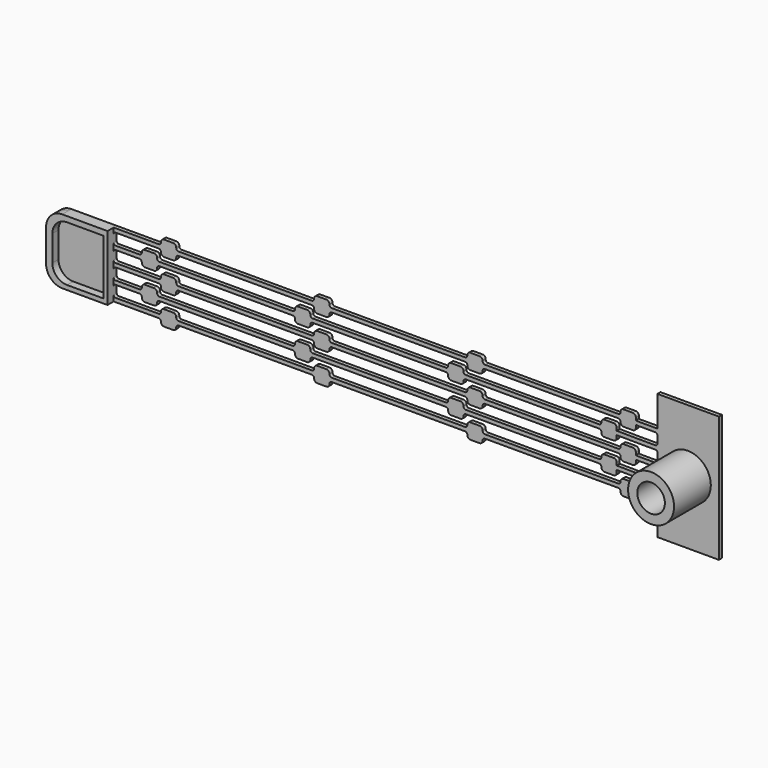
from build123d import *

# Parameters (mm, degrees)
F1_DEPTH = 0.25
F3_DEPTH = 0.5
F5_DEPTH = 0.5
F6_R     = 1.5
F6_R_2   = 0.9
F7_DEPTH = 3


# Not quite as in the source:
# - ends of sketch curves that miss each other by under 0.0002 mm in the source are joined


with BuildPart() as f1:
    # F0 (on Front) → F1 (new body)
    with BuildSketch(Plane.XZ):
        with BuildLine():
            Line((49.9212476134, 27.0172210783), (50.5212476134, 27.0172210783))
            ThreePointArc((50.5212476134, 27.0172210783), (50.6626689697, 27.075799722), (50.7212476134, 27.2172210783))
            Line((50.7212476134, 27.2172210783), (50.7212476134, 27.2422210783))
            ThreePointArc((50.7212476134, 27.2422210783), (50.7651815963, 27.3482870955), (50.8712476134, 27.3922210783))
            Line((50.8712476134, 27.3922210783), (51.1654019356, 27.3922210783))
            Line((51.1654019356, 27.3922210783), (57.8865653276, 27.3922210783))
            Line((57.8865653276, 27.3922210783), (59.1332476134, 27.3922210783))
            Line((59.1332476134, 27.3922210783), (59.5712476134, 27.3922210783))
            ThreePointArc((59.5712476134, 27.3922210783), (59.6773136306, 27.3482870955), (59.7212476134, 27.2422210783))
            Line((59.7212476134, 27.2422210783), (59.7212476134, 27.2172210783))
            ThreePointArc((59.7212476134, 27.2172210783), (59.7798262572, 27.075799722), (59.9212476134, 27.0172210783))
            Line((59.9212476134, 27.0172210783), (60.5212476134, 27.0172210783))
            ThreePointArc((60.5212476134, 27.0172210783), (60.6626689697, 27.075799722), (60.7212476134, 27.2172210783))
            Line((60.7212476134, 27.2172210783), (60.7212476134, 27.2422210783))
            ThreePointArc((60.7212476134, 27.2422210783), (60.7651815963, 27.3482870955), (60.8712476134, 27.3922210783))
            Line((60.8712476134, 27.3922210783), (61.1654019356, 27.3922210783))
            Line((61.1654019356, 27.3922210783), (67.8865653276, 27.3922210783))
            Line((67.8865653276, 27.3922210783), (69.1332476134, 27.3922210783))
            Line((69.1332476134, 27.3922210783), (69.5712476134, 27.3922210783))
            ThreePointArc((69.5712476134, 27.3922210783), (69.6773136306, 27.3482870955), (69.7212476134, 27.2422210783))
            Line((69.7212476134, 27.2422210783), (69.7212476134, 27.2172210783))
            ThreePointArc((69.7212476134, 27.2172210783), (69.7798262572, 27.075799722), (69.9212476134, 27.0172210783))
            Line((69.9212476134, 27.0172210783), (70.5212476134, 27.0172210783))
            ThreePointArc((70.5212476134, 27.0172210783), (70.6626689697, 27.075799722), (70.7212476134, 27.2172210783))
            Line((70.7212476134, 27.2172210783), (70.7212476134, 27.2422210783))
            ThreePointArc((70.7212476134, 27.2422210783), (70.7651815963, 27.3482870955), (70.8712476134, 27.3922210783))
            Line((70.8712476134, 27.3922210783), (71.1654019356, 27.3922210783))
            Line((71.1654019356, 27.3922210783), (77.8865653276, 27.3922210783))
            Line((77.8865653276, 27.3922210783), (79.1332476134, 27.3922210783))
            Line((79.1332476134, 27.3922210783), (79.5712476134, 27.3922210783))
            ThreePointArc((79.5712476134, 27.3922210783), (79.6773136306, 27.3482870955), (79.7212476134, 27.2422210783))
            Line((79.7212476134, 27.2422210783), (79.7212476134, 27.2172210783))
            ThreePointArc((79.7212476134, 27.2172210783), (79.7798262572, 27.075799722), (79.9212476134, 27.0172210783))
            Line((79.9212476134, 27.0172210783), (80.5212476134, 27.0172210783))
            ThreePointArc((80.5212476134, 27.0172210783), (80.6626689697, 27.075799722), (80.7212476134, 27.2172210783))
            Line((80.7212476134, 27.2172210783), (80.7212476134, 27.2422210783))
            Line((80.7212476134, 27.2422210783), (80.7212476134, 27.3922210783))
            Line((80.7212476134, 27.3922210783), (80.8795653284, 27.3786683083))
            Line((80.8795653284, 27.3786683083), (82.1295653284, 27.3786683083))
            Line((82.1295653284, 27.3786683083), (82.1295653284, 25.3928024322))
            Line((82.1295653284, 25.3928024322), (86.1411392689, 25.3928024322))
            Line((86.1411392689, 25.3928024322), (86.1411392689, 27.3786683083))
            Line((86.1411392689, 27.3786683083), (86.1411392689, 28.4439172033))
            Line((86.1411392689, 28.4439172033), (86.1411392689, 30.5634194132))
            Line((86.1411392689, 30.5634194132), (86.1411392689, 31.6286683083))
            Line((86.1411392689, 31.6286683083), (86.1411392689, 33.6259715259))
            Line((86.1411392689, 33.6259715259), (82.1295653284, 33.6259715259))
            Line((82.1295653284, 33.6259715259), (82.1295653284, 31.6286683083))
            Line((82.1295653284, 31.6286683083), (80.8795653284, 31.6286683083))
            Line((80.8795653284, 31.6286683083), (80.7212476134, 31.6422210783))
            Line((80.7212476134, 31.6422210783), (80.7212476134, 31.7922210783))
            Line((80.7212476134, 31.7922210783), (80.7212476134, 31.8172210783))
            ThreePointArc((80.7212476134, 31.8172210783), (80.6626689697, 31.9586424345), (80.5212476134, 32.0172210783))
            Line((80.5212476134, 32.0172210783), (79.9212476134, 32.0172210783))
            ThreePointArc((79.9212476134, 32.0172210783), (79.7798262572, 31.9586424345), (79.7212476134, 31.8172210783))
            Line((79.7212476134, 31.8172210783), (79.7212476134, 31.7922210783))
            ThreePointArc((79.7212476134, 31.7922210783), (79.6773136306, 31.6861550611), (79.5712476134, 31.6422210783))
            Line((79.5712476134, 31.6422210783), (79.1332476134, 31.6422210783))
            Line((79.1332476134, 31.6422210783), (77.8865653276, 31.6422210783))
            Line((77.8865653276, 31.6422210783), (71.1654019356, 31.6422210783))
            Line((71.1654019356, 31.6422210783), (70.8712476134, 31.6422210783))
            ThreePointArc((70.8712476134, 31.6422210783), (70.7651815963, 31.6861550611), (70.7212476134, 31.7922210783))
            Line((70.7212476134, 31.7922210783), (70.7212476134, 31.8172210783))
            ThreePointArc((70.7212476134, 31.8172210783), (70.6626689697, 31.9586424345), (70.5212476134, 32.0172210783))
            Line((70.5212476134, 32.0172210783), (69.9212476134, 32.0172210783))
            ThreePointArc((69.9212476134, 32.0172210783), (69.7798262572, 31.9586424345), (69.7212476134, 31.8172210783))
            Line((69.7212476134, 31.8172210783), (69.7212476134, 31.7922210783))
            ThreePointArc((69.7212476134, 31.7922210783), (69.6773136306, 31.6861550611), (69.5712476134, 31.6422210783))
            Line((69.5712476134, 31.6422210783), (69.1332476134, 31.6422210783))
            Line((69.1332476134, 31.6422210783), (67.8865653276, 31.6422210783))
            Line((67.8865653276, 31.6422210783), (61.1654019356, 31.6422210783))
            Line((61.1654019356, 31.6422210783), (60.8712476134, 31.6422210783))
            ThreePointArc((60.8712476134, 31.6422210783), (60.7651815963, 31.6861550611), (60.7212476134, 31.7922210783))
            Line((60.7212476134, 31.7922210783), (60.7212476134, 31.8172210783))
            ThreePointArc((60.7212476134, 31.8172210783), (60.6626689697, 31.9586424345), (60.5212476134, 32.0172210783))
            Line((60.5212476134, 32.0172210783), (59.9212476134, 32.0172210783))
            ThreePointArc((59.9212476134, 32.0172210783), (59.7798262572, 31.9586424345), (59.7212476134, 31.8172210783))
            Line((59.7212476134, 31.8172210783), (59.7212476134, 31.7922210783))
            ThreePointArc((59.7212476134, 31.7922210783), (59.6773136306, 31.6861550611), (59.5712476134, 31.6422210783))
            Line((59.5712476134, 31.6422210783), (59.1332476134, 31.6422210783))
            Line((59.1332476134, 31.6422210783), (57.8865653276, 31.6422210783))
            Line((57.8865653276, 31.6422210783), (51.1654019356, 31.6422210783))
            Line((51.1654019356, 31.6422210783), (50.8712476134, 31.6422210783))
            ThreePointArc((50.8712476134, 31.6422210783), (50.7651815963, 31.6861550611), (50.7212476134, 31.7922210783))
            Line((50.7212476134, 31.7922210783), (50.7212476134, 31.8172210783))
            ThreePointArc((50.7212476134, 31.8172210783), (50.6626689697, 31.9586424345), (50.5212476134, 32.0172210783))
            Line((50.5212476134, 32.0172210783), (49.9212476134, 32.0172210783))
            ThreePointArc((49.9212476134, 32.0172210783), (49.7798262572, 31.9586424345), (49.7212476134, 31.8172210783))
            Line((49.7212476134, 31.8172210783), (49.7212476134, 31.7922210783))
            ThreePointArc((49.7212476134, 31.7922210783), (49.6773136306, 31.6861550611), (49.5712476134, 31.6422210783))
            Line((49.5712476134, 31.6422210783), (49.1332476134, 31.6422210783))
            Line((49.1332476134, 31.6422210783), (47.8865653276, 31.6422210783))
            Line((47.8865653276, 31.6422210783), (43.6902402822, 31.6422210783))
            ThreePointArc((43.6902402822, 31.6422210783), (42.9369955648, 31.3302169006), (42.6249913871, 30.5769721832))
            Line((42.6249913871, 30.5769721832), (42.6249913871, 28.4574699733))
            ThreePointArc((42.6249913871, 28.4574699733), (42.9369955648, 27.704225256), (43.6902402822, 27.3922210783))
            Line((43.6902402822, 27.3922210783), (47.8865653276, 27.3922210783))
            Line((47.8865653276, 27.3922210783), (49.1332476134, 27.3922210783))
            Line((49.1332476134, 27.3922210783), (49.5712476134, 27.3922210783))
            ThreePointArc((49.5712476134, 27.3922210783), (49.6773136306, 27.3482870955), (49.7212476134, 27.2422210783))
            Line((49.7212476134, 27.2422210783), (49.7212476134, 27.2172210783))
            ThreePointArc((49.7212476134, 27.2172210783), (49.7798262572, 27.075799722), (49.9212476134, 27.0172210783))
        make_face()
        with BuildLine():
            ThreePointArc((50.7212476134, 27.8172210783), (50.6626689697, 27.9586424345), (50.5212476134, 28.0172210783))
            Line((50.5212476134, 28.0172210783), (49.9212476134, 28.0172210783))
            ThreePointArc((49.9212476134, 28.0172210783), (49.7798262572, 27.9586424345), (49.7212476134, 27.8172210783))
            Line((49.7212476134, 27.8172210783), (49.7212476134, 27.7922210783))
            ThreePointArc((49.7212476134, 27.7922210783), (49.6773136306, 27.6861550611), (49.5712476134, 27.6422210783))
            Line((49.5712476134, 27.6422210783), (49.1332476134, 27.6422210783))
            Line((49.1332476134, 27.6422210783), (47.8865653276, 27.6422210783))
            Line((47.8865653276, 27.6422210783), (46.7647824857, 27.6422210783))
            ThreePointArc((46.7647824857, 27.6422210783), (46.6741192638, 27.6797750144), (46.6365653276, 27.7704382363))
            Line((46.6365653276, 27.7704382363), (46.6365653276, 28.2640039202))
            ThreePointArc((46.6365653276, 28.2640039202), (46.6741192638, 28.3546671421), (46.7647824857, 28.3922210783))
            Line((46.7647824857, 28.3922210783), (47.8865653276, 28.3922210783))
            Line((47.8865653276, 28.3922210783), (48.3212476134, 28.3922210783))
            ThreePointArc((48.3212476134, 28.3922210783), (48.4273136306, 28.3482870955), (48.4712476134, 28.2422210783))
            Line((48.4712476134, 28.2422210783), (48.4712476134, 28.2172210783))
            ThreePointArc((48.4712476134, 28.2172210783), (48.5298262572, 28.075799722), (48.6712476134, 28.0172210783))
            Line((48.6712476134, 28.0172210783), (49.2712476134, 28.0172210783))
            ThreePointArc((49.2712476134, 28.0172210783), (49.4126689697, 28.075799722), (49.4712476134, 28.2172210783))
            Line((49.4712476134, 28.2172210783), (49.4712476134, 28.2422210783))
            ThreePointArc((49.4712476134, 28.2422210783), (49.5151815963, 28.3482870955), (49.6212476134, 28.3922210783))
            Line((49.6212476134, 28.3922210783), (51.1654019356, 28.3922210783))
            Line((51.1654019356, 28.3922210783), (57.8865653276, 28.3922210783))
            Line((57.8865653276, 28.3922210783), (58.3212476134, 28.3922210783))
            ThreePointArc((58.3212476134, 28.3922210783), (58.4273136306, 28.3482870955), (58.4712476134, 28.2422210783))
            Line((58.4712476134, 28.2422210783), (58.4712476134, 28.2172210783))
            ThreePointArc((58.4712476134, 28.2172210783), (58.5298262572, 28.075799722), (58.6712476134, 28.0172210783))
            Line((58.6712476134, 28.0172210783), (59.2712476134, 28.0172210783))
            ThreePointArc((59.2712476134, 28.0172210783), (59.4126689697, 28.075799722), (59.4712476134, 28.2172210783))
            Line((59.4712476134, 28.2172210783), (59.4712476134, 28.2422210783))
            ThreePointArc((59.4712476134, 28.2422210783), (59.5151815963, 28.3482870955), (59.6212476134, 28.3922210783))
            Line((59.6212476134, 28.3922210783), (61.1654019356, 28.3922210783))
            Line((61.1654019356, 28.3922210783), (67.8865653276, 28.3922210783))
            Line((67.8865653276, 28.3922210783), (68.3212476134, 28.3922210783))
            ThreePointArc((68.3212476134, 28.3922210783), (68.4273136306, 28.3482870955), (68.4712476134, 28.2422210783))
            Line((68.4712476134, 28.2422210783), (68.4712476134, 28.2172210783))
            ThreePointArc((68.4712476134, 28.2172210783), (68.5298262572, 28.075799722), (68.6712476134, 28.0172210783))
            Line((68.6712476134, 28.0172210783), (69.2712476134, 28.0172210783))
            ThreePointArc((69.2712476134, 28.0172210783), (69.4126689697, 28.075799722), (69.4712476134, 28.2172210783))
            Line((69.4712476134, 28.2172210783), (69.4712476134, 28.2422210783))
            ThreePointArc((69.4712476134, 28.2422210783), (69.5151815963, 28.3482870955), (69.6212476134, 28.3922210783))
            Line((69.6212476134, 28.3922210783), (71.1654019356, 28.3922210783))
            Line((71.1654019356, 28.3922210783), (77.8865653276, 28.3922210783))
            Line((77.8865653276, 28.3922210783), (78.3212476134, 28.3922210783))
            ThreePointArc((78.3212476134, 28.3922210783), (78.4273136306, 28.3482870955), (78.4712476134, 28.2422210783))
            Line((78.4712476134, 28.2422210783), (78.4712476134, 28.2172210783))
            ThreePointArc((78.4712476134, 28.2172210783), (78.5298262572, 28.075799722), (78.6712476134, 28.0172210783))
            Line((78.6712476134, 28.0172210783), (79.2712476134, 28.0172210783))
            ThreePointArc((79.2712476134, 28.0172210783), (79.4126689697, 28.075799722), (79.4712476134, 28.2172210783))
            Line((79.4712476134, 28.2172210783), (79.4712476134, 28.2422210783))
            Line((79.4712476134, 28.2422210783), (79.4712476134, 28.3922210783))
            Line((79.4712476134, 28.3922210783), (80.8795653284, 28.3786683083))
            Line((80.8795653284, 28.3786683083), (82.0013481703, 28.3786683083))
            ThreePointArc((82.0013481703, 28.3786683083), (82.0920113922, 28.3411143721), (82.1295653284, 28.2504511502))
            Line((82.1295653284, 28.2504511502), (82.1295653284, 27.7568854663))
            ThreePointArc((82.1295653284, 27.7568854663), (82.0920113922, 27.6662222444), (82.0013481703, 27.6286683083))
            Line((82.0013481703, 27.6286683083), (80.8795653284, 27.6286683083))
            Line((80.8795653284, 27.6286683083), (80.7212476134, 27.6422210783))
            Line((80.7212476134, 27.6422210783), (80.7212476134, 27.7922210783))
            Line((80.7212476134, 27.7922210783), (80.7212476134, 27.8172210783))
            ThreePointArc((80.7212476134, 27.8172210783), (80.6626689697, 27.9586424345), (80.5212476134, 28.0172210783))
            Line((80.5212476134, 28.0172210783), (79.9212476134, 28.0172210783))
            ThreePointArc((79.9212476134, 28.0172210783), (79.7798262572, 27.9586424345), (79.7212476134, 27.8172210783))
            Line((79.7212476134, 27.8172210783), (79.7212476134, 27.7922210783))
            ThreePointArc((79.7212476134, 27.7922210783), (79.6773136306, 27.6861550611), (79.5712476134, 27.6422210783))
            Line((79.5712476134, 27.6422210783), (79.1332476134, 27.6422210783))
            Line((79.1332476134, 27.6422210783), (77.8865653276, 27.6422210783))
            Line((77.8865653276, 27.6422210783), (71.1654019356, 27.6422210783))
            Line((71.1654019356, 27.6422210783), (70.8712476134, 27.6422210783))
            ThreePointArc((70.8712476134, 27.6422210783), (70.7651815963, 27.6861550611), (70.7212476134, 27.7922210783))
            Line((70.7212476134, 27.7922210783), (70.7212476134, 27.8172210783))
            ThreePointArc((70.7212476134, 27.8172210783), (70.6626689697, 27.9586424345), (70.5212476134, 28.0172210783))
            Line((70.5212476134, 28.0172210783), (69.9212476134, 28.0172210783))
            ThreePointArc((69.9212476134, 28.0172210783), (69.7798262572, 27.9586424345), (69.7212476134, 27.8172210783))
            Line((69.7212476134, 27.8172210783), (69.7212476134, 27.7922210783))
            ThreePointArc((69.7212476134, 27.7922210783), (69.6773136306, 27.6861550611), (69.5712476134, 27.6422210783))
            Line((69.5712476134, 27.6422210783), (69.1332476134, 27.6422210783))
            Line((69.1332476134, 27.6422210783), (67.8865653276, 27.6422210783))
            Line((67.8865653276, 27.6422210783), (61.1654019356, 27.6422210783))
            Line((61.1654019356, 27.6422210783), (60.8712476134, 27.6422210783))
            ThreePointArc((60.8712476134, 27.6422210783), (60.7651815963, 27.6861550611), (60.7212476134, 27.7922210783))
            Line((60.7212476134, 27.7922210783), (60.7212476134, 27.8172210783))
            ThreePointArc((60.7212476134, 27.8172210783), (60.6626689697, 27.9586424345), (60.5212476134, 28.0172210783))
            Line((60.5212476134, 28.0172210783), (59.9212476134, 28.0172210783))
            ThreePointArc((59.9212476134, 28.0172210783), (59.7798262572, 27.9586424345), (59.7212476134, 27.8172210783))
            Line((59.7212476134, 27.8172210783), (59.7212476134, 27.7922210783))
            ThreePointArc((59.7212476134, 27.7922210783), (59.6773136306, 27.6861550611), (59.5712476134, 27.6422210783))
            Line((59.5712476134, 27.6422210783), (59.1332476134, 27.6422210783))
            Line((59.1332476134, 27.6422210783), (57.8865653276, 27.6422210783))
            Line((57.8865653276, 27.6422210783), (51.1654019356, 27.6422210783))
            Line((51.1654019356, 27.6422210783), (50.8712476134, 27.6422210783))
            ThreePointArc((50.8712476134, 27.6422210783), (50.7651815963, 27.6861550611), (50.7212476134, 27.7922210783))
            Line((50.7212476134, 27.7922210783), (50.7212476134, 27.8172210783))
        make_face(mode=Mode.SUBTRACT)
        with BuildLine():
            Line((48.3212476134, 28.6422210783), (47.8865653276, 28.6422210783))
            Line((47.8865653276, 28.6422210783), (46.7647824857, 28.6422210783))
            ThreePointArc((46.7647824857, 28.6422210783), (46.6741192638, 28.6797750144), (46.6365653276, 28.7704382363))
            Line((46.6365653276, 28.7704382363), (46.6365653276, 29.2640039202))
            ThreePointArc((46.6365653276, 29.2640039202), (46.6741192638, 29.3546671421), (46.7647824857, 29.3922210783))
            Line((46.7647824857, 29.3922210783), (47.8865653276, 29.3922210783))
            Line((47.8865653276, 29.3922210783), (49.1332476134, 29.3922210783))
            Line((49.1332476134, 29.3922210783), (49.5712476134, 29.3922210783))
            ThreePointArc((49.5712476134, 29.3922210783), (49.6773136306, 29.3482870955), (49.7212476134, 29.2422210783))
            Line((49.7212476134, 29.2422210783), (49.7212476134, 29.2172210783))
            ThreePointArc((49.7212476134, 29.2172210783), (49.7798262572, 29.075799722), (49.9212476134, 29.0172210783))
            Line((49.9212476134, 29.0172210783), (50.5212476134, 29.0172210783))
            ThreePointArc((50.5212476134, 29.0172210783), (50.6626689697, 29.075799722), (50.7212476134, 29.2172210783))
            Line((50.7212476134, 29.2172210783), (50.7212476134, 29.2422210783))
            ThreePointArc((50.7212476134, 29.2422210783), (50.7651815963, 29.3482870955), (50.8712476134, 29.3922210783))
            Line((50.8712476134, 29.3922210783), (51.1654019356, 29.3922210783))
            Line((51.1654019356, 29.3922210783), (57.8865653276, 29.3922210783))
            Line((57.8865653276, 29.3922210783), (59.1332476134, 29.3922210783))
            Line((59.1332476134, 29.3922210783), (59.5712476134, 29.3922210783))
            ThreePointArc((59.5712476134, 29.3922210783), (59.6773136306, 29.3482870955), (59.7212476134, 29.2422210783))
            Line((59.7212476134, 29.2422210783), (59.7212476134, 29.2172210783))
            ThreePointArc((59.7212476134, 29.2172210783), (59.7798262572, 29.075799722), (59.9212476134, 29.0172210783))
            Line((59.9212476134, 29.0172210783), (60.5212476134, 29.0172210783))
            ThreePointArc((60.5212476134, 29.0172210783), (60.6626689697, 29.075799722), (60.7212476134, 29.2172210783))
            Line((60.7212476134, 29.2172210783), (60.7212476134, 29.2422210783))
            ThreePointArc((60.7212476134, 29.2422210783), (60.7651815963, 29.3482870955), (60.8712476134, 29.3922210783))
            Line((60.8712476134, 29.3922210783), (61.1654019356, 29.3922210783))
            Line((61.1654019356, 29.3922210783), (67.8865653276, 29.3922210783))
            Line((67.8865653276, 29.3922210783), (69.1332476134, 29.3922210783))
            Line((69.1332476134, 29.3922210783), (69.5712476134, 29.3922210783))
            ThreePointArc((69.5712476134, 29.3922210783), (69.6773136306, 29.3482870955), (69.7212476134, 29.2422210783))
            Line((69.7212476134, 29.2422210783), (69.7212476134, 29.2172210783))
            ThreePointArc((69.7212476134, 29.2172210783), (69.7798262572, 29.075799722), (69.9212476134, 29.0172210783))
            Line((69.9212476134, 29.0172210783), (70.5212476134, 29.0172210783))
            ThreePointArc((70.5212476134, 29.0172210783), (70.6626689697, 29.075799722), (70.7212476134, 29.2172210783))
            Line((70.7212476134, 29.2172210783), (70.7212476134, 29.2422210783))
            ThreePointArc((70.7212476134, 29.2422210783), (70.7651815963, 29.3482870955), (70.8712476134, 29.3922210783))
            Line((70.8712476134, 29.3922210783), (71.1654019356, 29.3922210783))
            Line((71.1654019356, 29.3922210783), (77.8865653276, 29.3922210783))
            Line((77.8865653276, 29.3922210783), (79.1332476134, 29.3922210783))
            Line((79.1332476134, 29.3922210783), (79.5712476134, 29.3922210783))
            ThreePointArc((79.5712476134, 29.3922210783), (79.6773136306, 29.3482870955), (79.7212476134, 29.2422210783))
            Line((79.7212476134, 29.2422210783), (79.7212476134, 29.2172210783))
            ThreePointArc((79.7212476134, 29.2172210783), (79.7798262572, 29.075799722), (79.9212476134, 29.0172210783))
            Line((79.9212476134, 29.0172210783), (80.5212476134, 29.0172210783))
            ThreePointArc((80.5212476134, 29.0172210783), (80.6626689697, 29.075799722), (80.7212476134, 29.2172210783))
            Line((80.7212476134, 29.2172210783), (80.7212476134, 29.2422210783))
            Line((80.7212476134, 29.2422210783), (80.7212476134, 29.3922210783))
            Line((80.7212476134, 29.3922210783), (80.8795653284, 29.3786683083))
            Line((80.8795653284, 29.3786683083), (82.0013481703, 29.3786683083))
            ThreePointArc((82.0013481703, 29.3786683083), (82.0920113922, 29.3411143721), (82.1295653284, 29.2504511502))
            Line((82.1295653284, 29.2504511502), (82.1295653284, 28.7568854663))
            ThreePointArc((82.1295653284, 28.7568854663), (82.0920113922, 28.6662222444), (82.0013481703, 28.6286683083))
            Line((82.0013481703, 28.6286683083), (80.8795653284, 28.6286683083))
            Line((80.8795653284, 28.6286683083), (79.4712476134, 28.6422210783))
            Line((79.4712476134, 28.6422210783), (79.4712476134, 28.7922210783))
            Line((79.4712476134, 28.7922210783), (79.4712476134, 28.8172210783))
            ThreePointArc((79.4712476134, 28.8172210783), (79.4126689697, 28.9586424345), (79.2712476134, 29.0172210783))
            Line((79.2712476134, 29.0172210783), (78.6712476134, 29.0172210783))
            ThreePointArc((78.6712476134, 29.0172210783), (78.5298262572, 28.9586424345), (78.4712476134, 28.8172210783))
            Line((78.4712476134, 28.8172210783), (78.4712476134, 28.7922210783))
            ThreePointArc((78.4712476134, 28.7922210783), (78.4273136306, 28.6861550611), (78.3212476134, 28.6422210783))
            Line((78.3212476134, 28.6422210783), (77.8865653276, 28.6422210783))
            Line((77.8865653276, 28.6422210783), (71.1654019356, 28.6422210783))
            Line((71.1654019356, 28.6422210783), (69.6212476134, 28.6422210783))
            ThreePointArc((69.6212476134, 28.6422210783), (69.5151815963, 28.6861550611), (69.4712476134, 28.7922210783))
            Line((69.4712476134, 28.7922210783), (69.4712476134, 28.8172210783))
            ThreePointArc((69.4712476134, 28.8172210783), (69.4126689697, 28.9586424345), (69.2712476134, 29.0172210783))
            Line((69.2712476134, 29.0172210783), (68.6712476134, 29.0172210783))
            ThreePointArc((68.6712476134, 29.0172210783), (68.5298262572, 28.9586424345), (68.4712476134, 28.8172210783))
            Line((68.4712476134, 28.8172210783), (68.4712476134, 28.7922210783))
            ThreePointArc((68.4712476134, 28.7922210783), (68.4273136306, 28.6861550611), (68.3212476134, 28.6422210783))
            Line((68.3212476134, 28.6422210783), (67.8865653276, 28.6422210783))
            Line((67.8865653276, 28.6422210783), (61.1654019356, 28.6422210783))
            Line((61.1654019356, 28.6422210783), (59.6212476134, 28.6422210783))
            ThreePointArc((59.6212476134, 28.6422210783), (59.5151815963, 28.6861550611), (59.4712476134, 28.7922210783))
            Line((59.4712476134, 28.7922210783), (59.4712476134, 28.8172210783))
            ThreePointArc((59.4712476134, 28.8172210783), (59.4126689697, 28.9586424345), (59.2712476134, 29.0172210783))
            Line((59.2712476134, 29.0172210783), (58.6712476134, 29.0172210783))
            ThreePointArc((58.6712476134, 29.0172210783), (58.5298262572, 28.9586424345), (58.4712476134, 28.8172210783))
            Line((58.4712476134, 28.8172210783), (58.4712476134, 28.7922210783))
            ThreePointArc((58.4712476134, 28.7922210783), (58.4273136306, 28.6861550611), (58.3212476134, 28.6422210783))
            Line((58.3212476134, 28.6422210783), (57.8865653276, 28.6422210783))
            Line((57.8865653276, 28.6422210783), (51.1654019356, 28.6422210783))
            Line((51.1654019356, 28.6422210783), (49.6212476134, 28.6422210783))
            ThreePointArc((49.6212476134, 28.6422210783), (49.5151815963, 28.6861550611), (49.4712476134, 28.7922210783))
            Line((49.4712476134, 28.7922210783), (49.4712476134, 28.8172210783))
            ThreePointArc((49.4712476134, 28.8172210783), (49.4126689697, 28.9586424345), (49.2712476134, 29.0172210783))
            Line((49.2712476134, 29.0172210783), (48.6712476134, 29.0172210783))
            ThreePointArc((48.6712476134, 29.0172210783), (48.5298262572, 28.9586424345), (48.4712476134, 28.8172210783))
            Line((48.4712476134, 28.8172210783), (48.4712476134, 28.7922210783))
            ThreePointArc((48.4712476134, 28.7922210783), (48.4273136306, 28.6861550611), (48.3212476134, 28.6422210783))
        make_face(mode=Mode.SUBTRACT)
        with BuildLine():
            ThreePointArc((50.7212476134, 29.8172210783), (50.6626689697, 29.9586424345), (50.5212476134, 30.0172210783))
            Line((50.5212476134, 30.0172210783), (49.9212476134, 30.0172210783))
            ThreePointArc((49.9212476134, 30.0172210783), (49.7798262572, 29.9586424345), (49.7212476134, 29.8172210783))
            Line((49.7212476134, 29.8172210783), (49.7212476134, 29.7922210783))
            ThreePointArc((49.7212476134, 29.7922210783), (49.6773136306, 29.6861550611), (49.5712476134, 29.6422210783))
            Line((49.5712476134, 29.6422210783), (49.1332476134, 29.6422210783))
            Line((49.1332476134, 29.6422210783), (47.8865653276, 29.6422210783))
            Line((47.8865653276, 29.6422210783), (46.7647824857, 29.6422210783))
            ThreePointArc((46.7647824857, 29.6422210783), (46.6741192638, 29.6797750144), (46.6365653276, 29.7704382363))
            Line((46.6365653276, 29.7704382363), (46.6365653276, 30.2640039202))
            ThreePointArc((46.6365653276, 30.2640039202), (46.6741192638, 30.3546671421), (46.7647824857, 30.3922210783))
            Line((46.7647824857, 30.3922210783), (47.8865653276, 30.3922210783))
            Line((47.8865653276, 30.3922210783), (48.3212476134, 30.3922210783))
            ThreePointArc((48.3212476134, 30.3922210783), (48.4273136306, 30.3482870955), (48.4712476134, 30.2422210783))
            Line((48.4712476134, 30.2422210783), (48.4712476134, 30.2172210783))
            ThreePointArc((48.4712476134, 30.2172210783), (48.5298262572, 30.075799722), (48.6712476134, 30.0172210783))
            Line((48.6712476134, 30.0172210783), (49.2712476134, 30.0172210783))
            ThreePointArc((49.2712476134, 30.0172210783), (49.4126689697, 30.075799722), (49.4712476134, 30.2172210783))
            Line((49.4712476134, 30.2172210783), (49.4712476134, 30.2422210783))
            ThreePointArc((49.4712476134, 30.2422210783), (49.5151815963, 30.3482870955), (49.6212476134, 30.3922210783))
            Line((49.6212476134, 30.3922210783), (51.1654019356, 30.3922210783))
            Line((51.1654019356, 30.3922210783), (57.8865653276, 30.3922210783))
            Line((57.8865653276, 30.3922210783), (58.3212476134, 30.3922210783))
            ThreePointArc((58.3212476134, 30.3922210783), (58.4273136306, 30.3482870955), (58.4712476134, 30.2422210783))
            Line((58.4712476134, 30.2422210783), (58.4712476134, 30.2172210783))
            ThreePointArc((58.4712476134, 30.2172210783), (58.5298262572, 30.075799722), (58.6712476134, 30.0172210783))
            Line((58.6712476134, 30.0172210783), (59.2712476134, 30.0172210783))
            ThreePointArc((59.2712476134, 30.0172210783), (59.4126689697, 30.075799722), (59.4712476134, 30.2172210783))
            Line((59.4712476134, 30.2172210783), (59.4712476134, 30.2422210783))
            ThreePointArc((59.4712476134, 30.2422210783), (59.5151815963, 30.3482870955), (59.6212476134, 30.3922210783))
            Line((59.6212476134, 30.3922210783), (61.1654019356, 30.3922210783))
            Line((61.1654019356, 30.3922210783), (67.8865653276, 30.3922210783))
            Line((67.8865653276, 30.3922210783), (68.3212476134, 30.3922210783))
            ThreePointArc((68.3212476134, 30.3922210783), (68.4273136306, 30.3482870955), (68.4712476134, 30.2422210783))
            Line((68.4712476134, 30.2422210783), (68.4712476134, 30.2172210783))
            ThreePointArc((68.4712476134, 30.2172210783), (68.5298262572, 30.075799722), (68.6712476134, 30.0172210783))
            Line((68.6712476134, 30.0172210783), (69.2712476134, 30.0172210783))
            ThreePointArc((69.2712476134, 30.0172210783), (69.4126689697, 30.075799722), (69.4712476134, 30.2172210783))
            Line((69.4712476134, 30.2172210783), (69.4712476134, 30.2422210783))
            ThreePointArc((69.4712476134, 30.2422210783), (69.5151815963, 30.3482870955), (69.6212476134, 30.3922210783))
            Line((69.6212476134, 30.3922210783), (71.1654019356, 30.3922210783))
            Line((71.1654019356, 30.3922210783), (77.8865653276, 30.3922210783))
            Line((77.8865653276, 30.3922210783), (78.3212476134, 30.3922210783))
            ThreePointArc((78.3212476134, 30.3922210783), (78.4273136306, 30.3482870955), (78.4712476134, 30.2422210783))
            Line((78.4712476134, 30.2422210783), (78.4712476134, 30.2172210783))
            ThreePointArc((78.4712476134, 30.2172210783), (78.5298262572, 30.075799722), (78.6712476134, 30.0172210783))
            Line((78.6712476134, 30.0172210783), (79.2712476134, 30.0172210783))
            ThreePointArc((79.2712476134, 30.0172210783), (79.4126689697, 30.075799722), (79.4712476134, 30.2172210783))
            Line((79.4712476134, 30.2172210783), (79.4712476134, 30.2422210783))
            Line((79.4712476134, 30.2422210783), (79.4712476134, 30.3922210783))
            Line((79.4712476134, 30.3922210783), (80.8795653284, 30.3786683083))
            Line((80.8795653284, 30.3786683083), (82.0013481703, 30.3786683083))
            ThreePointArc((82.0013481703, 30.3786683083), (82.0920113922, 30.3411143721), (82.1295653284, 30.2504511502))
            Line((82.1295653284, 30.2504511502), (82.1295653284, 29.7568854663))
            ThreePointArc((82.1295653284, 29.7568854663), (82.0920113922, 29.6662222444), (82.0013481703, 29.6286683083))
            Line((82.0013481703, 29.6286683083), (80.8795653284, 29.6286683083))
            Line((80.8795653284, 29.6286683083), (80.7212476134, 29.6422210783))
            Line((80.7212476134, 29.6422210783), (80.7212476134, 29.7922210783))
            Line((80.7212476134, 29.7922210783), (80.7212476134, 29.8172210783))
            ThreePointArc((80.7212476134, 29.8172210783), (80.6626689697, 29.9586424345), (80.5212476134, 30.0172210783))
            Line((80.5212476134, 30.0172210783), (79.9212476134, 30.0172210783))
            ThreePointArc((79.9212476134, 30.0172210783), (79.7798262572, 29.9586424345), (79.7212476134, 29.8172210783))
            Line((79.7212476134, 29.8172210783), (79.7212476134, 29.7922210783))
            ThreePointArc((79.7212476134, 29.7922210783), (79.6773136306, 29.6861550611), (79.5712476134, 29.6422210783))
            Line((79.5712476134, 29.6422210783), (79.1332476134, 29.6422210783))
            Line((79.1332476134, 29.6422210783), (77.8865653276, 29.6422210783))
            Line((77.8865653276, 29.6422210783), (71.1654019356, 29.6422210783))
            Line((71.1654019356, 29.6422210783), (70.8712476134, 29.6422210783))
            ThreePointArc((70.8712476134, 29.6422210783), (70.7651815963, 29.6861550611), (70.7212476134, 29.7922210783))
            Line((70.7212476134, 29.7922210783), (70.7212476134, 29.8172210783))
            ThreePointArc((70.7212476134, 29.8172210783), (70.6626689697, 29.9586424345), (70.5212476134, 30.0172210783))
            Line((70.5212476134, 30.0172210783), (69.9212476134, 30.0172210783))
            ThreePointArc((69.9212476134, 30.0172210783), (69.7798262572, 29.9586424345), (69.7212476134, 29.8172210783))
            Line((69.7212476134, 29.8172210783), (69.7212476134, 29.7922210783))
            ThreePointArc((69.7212476134, 29.7922210783), (69.6773136306, 29.6861550611), (69.5712476134, 29.6422210783))
            Line((69.5712476134, 29.6422210783), (69.1332476134, 29.6422210783))
            Line((69.1332476134, 29.6422210783), (67.8865653276, 29.6422210783))
            Line((67.8865653276, 29.6422210783), (61.1654019356, 29.6422210783))
            Line((61.1654019356, 29.6422210783), (60.8712476134, 29.6422210783))
            ThreePointArc((60.8712476134, 29.6422210783), (60.7651815963, 29.6861550611), (60.7212476134, 29.7922210783))
            Line((60.7212476134, 29.7922210783), (60.7212476134, 29.8172210783))
            ThreePointArc((60.7212476134, 29.8172210783), (60.6626689697, 29.9586424345), (60.5212476134, 30.0172210783))
            Line((60.5212476134, 30.0172210783), (59.9212476134, 30.0172210783))
            ThreePointArc((59.9212476134, 30.0172210783), (59.7798262572, 29.9586424345), (59.7212476134, 29.8172210783))
            Line((59.7212476134, 29.8172210783), (59.7212476134, 29.7922210783))
            ThreePointArc((59.7212476134, 29.7922210783), (59.6773136306, 29.6861550611), (59.5712476134, 29.6422210783))
            Line((59.5712476134, 29.6422210783), (59.1332476134, 29.6422210783))
            Line((59.1332476134, 29.6422210783), (57.8865653276, 29.6422210783))
            Line((57.8865653276, 29.6422210783), (51.1654019356, 29.6422210783))
            Line((51.1654019356, 29.6422210783), (50.8712476134, 29.6422210783))
            ThreePointArc((50.8712476134, 29.6422210783), (50.7651815963, 29.6861550611), (50.7212476134, 29.7922210783))
            Line((50.7212476134, 29.7922210783), (50.7212476134, 29.8172210783))
        make_face(mode=Mode.SUBTRACT)
        with BuildLine():
            Line((48.3212476134, 30.6422210783), (47.8865653276, 30.6422210783))
            Line((47.8865653276, 30.6422210783), (46.7647824857, 30.6422210783))
            ThreePointArc((46.7647824857, 30.6422210783), (46.6741192638, 30.6797750144), (46.6365653276, 30.7704382363))
            Line((46.6365653276, 30.7704382363), (46.6365653276, 31.2640039202))
            ThreePointArc((46.6365653276, 31.2640039202), (46.6741192638, 31.3546671421), (46.7647824857, 31.3922210783))
            Line((46.7647824857, 31.3922210783), (47.8865653276, 31.3922210783))
            Line((47.8865653276, 31.3922210783), (49.1332476134, 31.3922210783))
            Line((49.1332476134, 31.3922210783), (49.5712476134, 31.3922210783))
            ThreePointArc((49.5712476134, 31.3922210783), (49.6773136306, 31.3482870955), (49.7212476134, 31.2422210783))
            Line((49.7212476134, 31.2422210783), (49.7212476134, 31.2172210783))
            ThreePointArc((49.7212476134, 31.2172210783), (49.7798262572, 31.075799722), (49.9212476134, 31.0172210783))
            Line((49.9212476134, 31.0172210783), (50.5212476134, 31.0172210783))
            ThreePointArc((50.5212476134, 31.0172210783), (50.6626689697, 31.075799722), (50.7212476134, 31.2172210783))
            Line((50.7212476134, 31.2172210783), (50.7212476134, 31.2422210783))
            ThreePointArc((50.7212476134, 31.2422210783), (50.7651815963, 31.3482870955), (50.8712476134, 31.3922210783))
            Line((50.8712476134, 31.3922210783), (51.1654019356, 31.3922210783))
            Line((51.1654019356, 31.3922210783), (57.8865653276, 31.3922210783))
            Line((57.8865653276, 31.3922210783), (59.1332476134, 31.3922210783))
            Line((59.1332476134, 31.3922210783), (59.5712476134, 31.3922210783))
            ThreePointArc((59.5712476134, 31.3922210783), (59.6773136306, 31.3482870955), (59.7212476134, 31.2422210783))
            Line((59.7212476134, 31.2422210783), (59.7212476134, 31.2172210783))
            ThreePointArc((59.7212476134, 31.2172210783), (59.7798262572, 31.075799722), (59.9212476134, 31.0172210783))
            Line((59.9212476134, 31.0172210783), (60.5212476134, 31.0172210783))
            ThreePointArc((60.5212476134, 31.0172210783), (60.6626689697, 31.075799722), (60.7212476134, 31.2172210783))
            Line((60.7212476134, 31.2172210783), (60.7212476134, 31.2422210783))
            ThreePointArc((60.7212476134, 31.2422210783), (60.7651815963, 31.3482870955), (60.8712476134, 31.3922210783))
            Line((60.8712476134, 31.3922210783), (61.1654019356, 31.3922210783))
            Line((61.1654019356, 31.3922210783), (67.8865653276, 31.3922210783))
            Line((67.8865653276, 31.3922210783), (69.1332476134, 31.3922210783))
            Line((69.1332476134, 31.3922210783), (69.5712476134, 31.3922210783))
            ThreePointArc((69.5712476134, 31.3922210783), (69.6773136306, 31.3482870955), (69.7212476134, 31.2422210783))
            Line((69.7212476134, 31.2422210783), (69.7212476134, 31.2172210783))
            ThreePointArc((69.7212476134, 31.2172210783), (69.7798262572, 31.075799722), (69.9212476134, 31.0172210783))
            Line((69.9212476134, 31.0172210783), (70.5212476134, 31.0172210783))
            ThreePointArc((70.5212476134, 31.0172210783), (70.6626689697, 31.075799722), (70.7212476134, 31.2172210783))
            Line((70.7212476134, 31.2172210783), (70.7212476134, 31.2422210783))
            ThreePointArc((70.7212476134, 31.2422210783), (70.7651815963, 31.3482870955), (70.8712476134, 31.3922210783))
            Line((70.8712476134, 31.3922210783), (71.1654019356, 31.3922210783))
            Line((71.1654019356, 31.3922210783), (77.8865653276, 31.3922210783))
            Line((77.8865653276, 31.3922210783), (79.1332476134, 31.3922210783))
            Line((79.1332476134, 31.3922210783), (79.5712476134, 31.3922210783))
            ThreePointArc((79.5712476134, 31.3922210783), (79.6773136306, 31.3482870955), (79.7212476134, 31.2422210783))
            Line((79.7212476134, 31.2422210783), (79.7212476134, 31.2172210783))
            ThreePointArc((79.7212476134, 31.2172210783), (79.7798262572, 31.075799722), (79.9212476134, 31.0172210783))
            Line((79.9212476134, 31.0172210783), (80.5212476134, 31.0172210783))
            ThreePointArc((80.5212476134, 31.0172210783), (80.6626689697, 31.075799722), (80.7212476134, 31.2172210783))
            Line((80.7212476134, 31.2172210783), (80.7212476134, 31.2422210783))
            Line((80.7212476134, 31.2422210783), (80.7212476134, 31.3922210783))
            Line((80.7212476134, 31.3922210783), (80.8795653284, 31.3786683083))
            Line((80.8795653284, 31.3786683083), (82.0013481703, 31.3786683083))
            ThreePointArc((82.0013481703, 31.3786683083), (82.0920113922, 31.3411143721), (82.1295653284, 31.2504511502))
            Line((82.1295653284, 31.2504511502), (82.1295653284, 30.7568854663))
            ThreePointArc((82.1295653284, 30.7568854663), (82.0920113922, 30.6662222444), (82.0013481703, 30.6286683083))
            Line((82.0013481703, 30.6286683083), (80.8795653284, 30.6286683083))
            Line((80.8795653284, 30.6286683083), (79.4712476134, 30.6422210783))
            Line((79.4712476134, 30.6422210783), (79.4712476134, 30.7922210783))
            Line((79.4712476134, 30.7922210783), (79.4712476134, 30.8172210783))
            ThreePointArc((79.4712476134, 30.8172210783), (79.4126689697, 30.9586424345), (79.2712476134, 31.0172210783))
            Line((79.2712476134, 31.0172210783), (78.6712476134, 31.0172210783))
            ThreePointArc((78.6712476134, 31.0172210783), (78.5298262572, 30.9586424345), (78.4712476134, 30.8172210783))
            Line((78.4712476134, 30.8172210783), (78.4712476134, 30.7922210783))
            ThreePointArc((78.4712476134, 30.7922210783), (78.4273136306, 30.6861550611), (78.3212476134, 30.6422210783))
            Line((78.3212476134, 30.6422210783), (77.8865653276, 30.6422210783))
            Line((77.8865653276, 30.6422210783), (71.1654019356, 30.6422210783))
            Line((71.1654019356, 30.6422210783), (69.6212476134, 30.6422210783))
            ThreePointArc((69.6212476134, 30.6422210783), (69.5151815963, 30.6861550611), (69.4712476134, 30.7922210783))
            Line((69.4712476134, 30.7922210783), (69.4712476134, 30.8172210783))
            ThreePointArc((69.4712476134, 30.8172210783), (69.4126689697, 30.9586424345), (69.2712476134, 31.0172210783))
            Line((69.2712476134, 31.0172210783), (68.6712476134, 31.0172210783))
            ThreePointArc((68.6712476134, 31.0172210783), (68.5298262572, 30.9586424345), (68.4712476134, 30.8172210783))
            Line((68.4712476134, 30.8172210783), (68.4712476134, 30.7922210783))
            ThreePointArc((68.4712476134, 30.7922210783), (68.4273136306, 30.6861550611), (68.3212476134, 30.6422210783))
            Line((68.3212476134, 30.6422210783), (67.8865653276, 30.6422210783))
            Line((67.8865653276, 30.6422210783), (61.1654019356, 30.6422210783))
            Line((61.1654019356, 30.6422210783), (59.6212476134, 30.6422210783))
            ThreePointArc((59.6212476134, 30.6422210783), (59.5151815963, 30.6861550611), (59.4712476134, 30.7922210783))
            Line((59.4712476134, 30.7922210783), (59.4712476134, 30.8172210783))
            ThreePointArc((59.4712476134, 30.8172210783), (59.4126689697, 30.9586424345), (59.2712476134, 31.0172210783))
            Line((59.2712476134, 31.0172210783), (58.6712476134, 31.0172210783))
            ThreePointArc((58.6712476134, 31.0172210783), (58.5298262572, 30.9586424345), (58.4712476134, 30.8172210783))
            Line((58.4712476134, 30.8172210783), (58.4712476134, 30.7922210783))
            ThreePointArc((58.4712476134, 30.7922210783), (58.4273136306, 30.6861550611), (58.3212476134, 30.6422210783))
            Line((58.3212476134, 30.6422210783), (57.8865653276, 30.6422210783))
            Line((57.8865653276, 30.6422210783), (51.1654019356, 30.6422210783))
            Line((51.1654019356, 30.6422210783), (49.6212476134, 30.6422210783))
            ThreePointArc((49.6212476134, 30.6422210783), (49.5151815963, 30.6861550611), (49.4712476134, 30.7922210783))
            Line((49.4712476134, 30.7922210783), (49.4712476134, 30.8172210783))
            ThreePointArc((49.4712476134, 30.8172210783), (49.4126689697, 30.9586424345), (49.2712476134, 31.0172210783))
            Line((49.2712476134, 31.0172210783), (48.6712476134, 31.0172210783))
            ThreePointArc((48.6712476134, 31.0172210783), (48.5298262572, 30.9586424345), (48.4712476134, 30.8172210783))
            Line((48.4712476134, 30.8172210783), (48.4712476134, 30.7922210783))
            ThreePointArc((48.4712476134, 30.7922210783), (48.4273136306, 30.6861550611), (48.3212476134, 30.6422210783))
        make_face(mode=Mode.SUBTRACT)
    extrude(amount=F1_DEPTH)

    # F2 (on face) → F3 (join)
    with BuildSketch(Plane.XZ.offset(0.25)):
        with BuildLine():
            Line((46.6365653276, 31.2640039202), (46.6365653276, 31.6422210783))
            Line((46.6365653276, 31.6422210783), (43.6902402822, 31.6422210783))
            Line((43.6902402822, 31.6422210783), (43.6797258529, 31.6422210783))
            ThreePointArc((43.6797258529, 31.6422210783), (42.933287461, 31.3264904518), (42.6249913871, 30.5769721832))
            Line((42.6249913871, 30.5769721832), (42.6249913871, 28.4574699733))
            ThreePointArc((42.6249913871, 28.4574699733), (42.933287461, 27.7079517048), (43.6797263651, 27.3922729653))
            Line((43.6797263651, 27.3922729653), (43.6902402822, 27.3922210783))
            Line((43.6902402822, 27.3922210783), (46.6365653276, 27.3922210783))
            Line((46.6365653276, 27.3922210783), (46.6365653276, 27.7704382363))
            Line((46.6365653276, 27.7704382363), (46.6365653276, 28.2640039202))
            Line((46.6365653276, 28.2640039202), (46.6365653276, 28.7704382363))
            Line((46.6365653276, 28.7704382363), (46.6365653276, 29.2640039202))
            Line((46.6365653276, 29.2640039202), (46.6365653276, 29.7704382363))
            Line((46.6365653276, 29.7704382363), (46.6365653276, 30.2640039202))
            Line((46.6365653276, 30.2640039202), (46.6365653276, 30.7704382363))
            Line((46.6365653276, 30.7704382363), (46.6365653276, 31.2640039202))
        make_face()
    extrude(amount=F3_DEPTH)

    # F4 (on face) → F5 (cut)
    with BuildSketch(Plane.XZ.offset(0.75)):
        with BuildLine():
            Line((46.3622398674, 27.6831910014), (46.3622398674, 31.2864722807))
            Line((46.3622398674, 31.2864722807), (43.9912102393, 31.2864722807))
            ThreePointArc((43.9912102393, 31.2864722807), (43.3149467205, 31.0063547595), (43.0348291993, 30.3300912407))
            Line((43.0348291993, 30.3300912407), (43.0348291993, 28.6395720414))
            ThreePointArc((43.0348291993, 28.6395720414), (43.3149467205, 27.9633085226), (43.9912102393, 27.6831910014))
            Line((43.9912102393, 27.6831910014), (46.3622398674, 27.6831910014))
        make_face()
    extrude(amount=-F5_DEPTH, mode=Mode.SUBTRACT)

    # F6 (on face) → F7 (join)
    with BuildSketch(Plane.XZ.offset(0.25)):
        with Locations((84.1165753306, 29.5036683083)):
            Circle(F6_R)
        with Locations((84.1165753306, 29.5036683083)):
            Circle(F6_R_2, mode=Mode.SUBTRACT)
    extrude(amount=F7_DEPTH)


solid = f1.part
